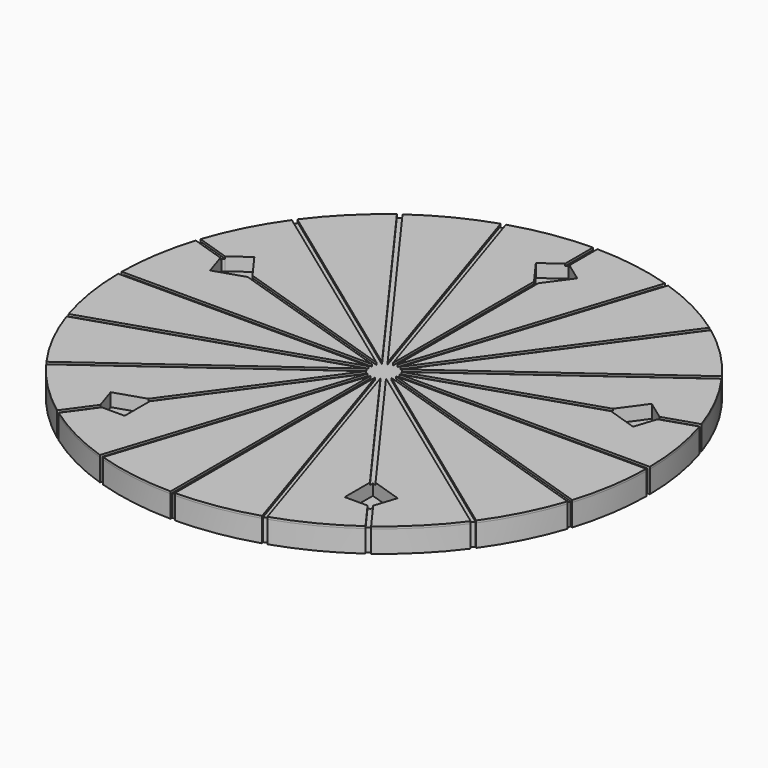
from build123d import *

# Parameters (mm, degrees)
F0_R            = 60
F1_DEPTH        = 5
F3_DEPTH        = 0.5
F4_W            = 5
F4_H            = 1
F5_DEPTH        = 5.501
F5_COPIES_COUNT = 20
F8_DEPTH        = 3
F9_R            = 5
F10_DEPTH       = 3


# Not quite as in the source:
# - a pattern or mirror of a feature is missing from the dataset's text; its kind, count and spacing are read off the source's solid


with BuildPart() as f1:
    # F0 (on Top) → F1 (new body)
    with BuildSketch(Plane.XY):
        Circle(F0_R)
    extrude(amount=F1_DEPTH)

    # F2 (on face) → F3 (join)
    with BuildSketch(Plane.XY.offset(5)):
        with BuildLine():
            ThreePointArc((59.9979166305, 0.5), (59.2613004357, 9.3860679024), (57.2159180728, 18.0648476078))
            Line((57.2159180728, 18.0648476078), (3.1568757573, 0.5))
            Line((3.1568757573, 0.5), (59.9979166305, 0.5))
        make_face()
        with BuildLine():
            ThreePointArc((56.9069010784, 19.0159041241), (53.4603914513, 27.2394299844), (48.8332268073, 34.8613820665))
            Line((48.8332268073, 34.8613820665), (2.847858763, 1.4510565163))
            Line((2.847858763, 1.4510565163), (56.9069010784, 19.0159041241))
        make_face()
        with BuildLine():
            ThreePointArc((48.245441555, 35.6703990609), (42.4264068712, 42.4264068712), (35.6703990609, 48.245441555))
            Line((35.6703990609, 48.245441555), (2.2600735107, 2.2600735107))
            Line((2.2600735107, 2.2600735107), (48.245441555, 35.6703990609))
        make_face()
        with BuildLine():
            ThreePointArc((34.8613820665, 48.8332268073), (27.2394299844, 53.4603914513), (19.0159041241, 56.9069010784))
            Line((19.0159041241, 56.9069010784), (1.4510565163, 2.847858763))
            Line((1.4510565163, 2.847858763), (34.8613820665, 48.8332268073))
        make_face()
        with BuildLine():
            ThreePointArc((18.0648476078, 57.2159180728), (9.3860679024, 59.2613004357), (0.5, 59.9979166305))
            Line((0.5, 59.9979166305), (0.5, 3.1568757573))
            Line((0.5, 3.1568757573), (18.0648476078, 57.2159180728))
        make_face()
        with BuildLine():
            ThreePointArc((-0.5, 59.9979166305), (-9.3860679024, 59.2613004357), (-18.0648476078, 57.2159180728))
            Line((-18.0648476078, 57.2159180728), (-0.5, 3.1568757573))
            Line((-0.5, 3.1568757573), (-0.5, 59.9979166305))
        make_face()
        with BuildLine():
            ThreePointArc((-19.0159041241, 56.9069010784), (-27.2394299844, 53.4603914513), (-34.8613820665, 48.8332268073))
            Line((-34.8613820665, 48.8332268073), (-1.4510565163, 2.847858763))
            Line((-1.4510565163, 2.847858763), (-19.0159041241, 56.9069010784))
        make_face()
        with BuildLine():
            ThreePointArc((-35.6703990609, 48.245441555), (-42.4264068712, 42.4264068712), (-48.245441555, 35.6703990609))
            Line((-48.245441555, 35.6703990609), (-2.2600735107, 2.2600735107))
            Line((-2.2600735107, 2.2600735107), (-35.6703990609, 48.245441555))
        make_face()
        with BuildLine():
            ThreePointArc((-48.8332268073, 34.8613820665), (-53.4603914513, 27.2394299844), (-56.9069010784, 19.0159041241))
            Line((-56.9069010784, 19.0159041241), (-2.847858763, 1.4510565163))
            Line((-2.847858763, 1.4510565163), (-48.8332268073, 34.8613820665))
        make_face()
        with BuildLine():
            ThreePointArc((-57.2159180728, 18.0648476078), (-59.2613004357, 9.3860679024), (-59.9979166305, 0.5))
            Line((-59.9979166305, 0.5), (-3.1568757573, 0.5))
            Line((-3.1568757573, 0.5), (-57.2159180728, 18.0648476078))
        make_face()
        with BuildLine():
            Line((-3.1568757573, -0.5), (-59.9979166305, -0.5))
            ThreePointArc((-59.9979166305, -0.5), (-59.2613004357, -9.3860679024), (-57.2159180728, -18.0648476078))
            Line((-57.2159180728, -18.0648476078), (-3.1568757573, -0.5))
        make_face()
        with BuildLine():
            Line((-2.847858763, -1.4510565163), (-56.9069010784, -19.0159041241))
            ThreePointArc((-56.9069010784, -19.0159041241), (-53.4603914513, -27.2394299844), (-48.8332268073, -34.8613820665))
            Line((-48.8332268073, -34.8613820665), (-2.847858763, -1.4510565163))
        make_face()
        with BuildLine():
            Line((-2.2600735107, -2.2600735107), (-48.245441555, -35.6703990609))
            ThreePointArc((-48.245441555, -35.6703990609), (-42.4264068712, -42.4264068712), (-35.6703990609, -48.245441555))
            Line((-35.6703990609, -48.245441555), (-2.2600735107, -2.2600735107))
        make_face()
        with BuildLine():
            Line((-1.4510565163, -2.847858763), (-34.8613820665, -48.8332268073))
            ThreePointArc((-34.8613820665, -48.8332268073), (-27.2394299844, -53.4603914513), (-19.0159041241, -56.9069010784))
            Line((-19.0159041241, -56.9069010784), (-1.4510565163, -2.847858763))
        make_face()
        with BuildLine():
            Line((-0.5, -3.1568757573), (-18.0648476078, -57.2159180728))
            ThreePointArc((-18.0648476078, -57.2159180728), (-9.3860679024, -59.2613004357), (-0.5, -59.9979166305))
            Line((-0.5, -59.9979166305), (-0.5, -3.1568757573))
        make_face()
        with BuildLine():
            Line((0.5, -3.1568757573), (0.5, -59.9979166305))
            ThreePointArc((0.5, -59.9979166305), (9.3860679024, -59.2613004357), (18.0648476078, -57.2159180728))
            Line((18.0648476078, -57.2159180728), (0.5, -3.1568757573))
        make_face()
        with BuildLine():
            Line((1.4510565163, -2.847858763), (19.0159041241, -56.9069010784))
            ThreePointArc((19.0159041241, -56.9069010784), (27.2394299844, -53.4603914513), (34.8613820665, -48.8332268073))
            Line((34.8613820665, -48.8332268073), (1.4510565163, -2.847858763))
        make_face()
        with BuildLine():
            Line((2.2600735107, -2.2600735107), (35.6703990609, -48.245441555))
            ThreePointArc((35.6703990609, -48.245441555), (42.4264068712, -42.4264068712), (48.245441555, -35.6703990609))
            Line((48.245441555, -35.6703990609), (2.2600735107, -2.2600735107))
        make_face()
        with BuildLine():
            Line((2.847858763, -1.4510565163), (48.8332268073, -34.8613820665))
            ThreePointArc((48.8332268073, -34.8613820665), (53.4603914513, -27.2394299844), (56.9069010784, -19.0159041241))
            Line((56.9069010784, -19.0159041241), (2.847858763, -1.4510565163))
        make_face()
        with BuildLine():
            Line((3.1568757573, -0.5), (57.2159180728, -18.0648476078))
            ThreePointArc((57.2159180728, -18.0648476078), (59.2613004357, -9.3860679024), (59.9979166305, -0.5))
            Line((59.9979166305, -0.5), (3.1568757573, -0.5))
        make_face()
    extrude(amount=F3_DEPTH)

    # F4 (on face) → F5 (cut, through all)
    with BuildSketch(Plane.XY.offset(5.5)):
        with Locations((-61.9979166305, 0)):
            Rectangle(F4_W, F4_H)
    f5 = extrude(amount=-F5_DEPTH, mode=Mode.SUBTRACT)

    # F5_copies: F5 ×20 about axis
    f5_copies_axis = Axis((0, 0, 0), (0, 0, 1))
    for i in range(1, F5_COPIES_COUNT):
        add(f5.rotate(f5_copies_axis, i * 360 / F5_COPIES_COUNT), mode=Mode.SUBTRACT)

    # F7 (on face) → F8 (cut)
    with BuildSketch(Plane.XY.offset(5.5)):
        Polygon((-4.7022820183, 49.0046763726), (0, 42.5325404176), (4.7022820183, 49.0046763726), (0, 52.4210842376), align=None)
        Polygon((-48.0593018491, 10.671141848), (-40.4508497187, 13.143277803), (-40.9508497187, 13.8314687632), (-49.3554137554, 16.562277157), (-49.8554137554, 16.199005893), align=None)
        Polygon((-49.3554137554, 16.562277157), (-40.9508497187, 13.8314687632), (-45.1531317371, 19.615413758), align=None)
        Polygon((45.1531317371, 19.615413758), (40.4508497187, 13.143277803), (48.0593018491, 10.671141848), (49.8554137554, 16.199005893), align=None)
        Polygon((-25, -42.4095480118), (-25, -34.4095480118), (-32.6084521304, -36.8816839668), (-30.812340224, -42.4095480118), align=None)
        Polygon((32.6084521304, -36.8816839668), (25, -34.4095480118), (25, -42.4095480118), (30.812340224, -42.4095480118), align=None)
    extrude(amount=-F8_DEPTH, mode=Mode.SUBTRACT)

    # F9 (on face) → F10 (cut)
    with BuildSketch(Plane(origin=(0, 0, 0), x_dir=(1, 0, 0), z_dir=(0, 0, -1))):
        with Locations((-24.0012126607, 31.9990904686)):
            Circle(F9_R)
        with Locations((-15.5012126607, -36.87427838)):
            Circle(F9_R)
        with Locations((39.9987873393, 0.3114665041)):
            Circle(F9_R)
    extrude(amount=-F10_DEPTH, mode=Mode.SUBTRACT)


solid = f1.part
